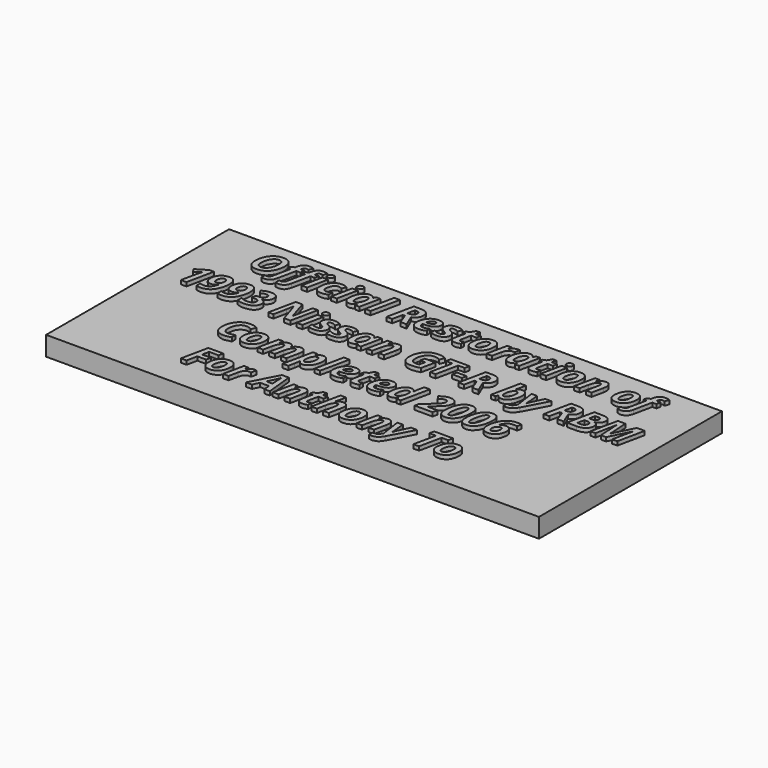
from build123d import *

# Parameters (mm, degrees)
F0_TEXT_SIZE = 12.5242310919
F2_DEPTH     = 7.62
F1_W         = 162.3541414738
F1_H         = 75.3404442221
F3_DEPTH     = 6.35


# Not quite as in the source:
# - Text() gives the source's letters only with a copy of the font that has no kerning and outlines rounded to 1/6400 em; it was checked with that copy


with BuildPart() as f2:
    # F0 (on Top) → F2 (new body)
    with BuildSketch(Plane.XY):
        with Locations((-64.2444132238, 17.4707429373)):
            Text('Official Restoration of', F0_TEXT_SIZE, font='Open Sans', font_style=FontStyle.BOLDITALIC, text_align=(TextAlign.LEFT, TextAlign.BOTTOM))
        with Locations((-74.0074427422, 0.4377886522)):
            Text('1993 Nissan GT-R by RBM', F0_TEXT_SIZE, font='Open Sans', font_style=FontStyle.BOLDITALIC, text_align=(TextAlign.LEFT, TextAlign.BOTTOM))
        with Locations((-47.9726973599, -16.5951656328)):
            Text('Completed 2006', F0_TEXT_SIZE, font='Open Sans', font_style=FontStyle.BOLDITALIC, text_align=(TextAlign.LEFT, TextAlign.BOTTOM))
        with Locations((-44.7183541871, -33.6281199178)):
            Text('For Anthony To', F0_TEXT_SIZE, font='Open Sans', font_style=FontStyle.BOLDITALIC, text_align=(TextAlign.LEFT, TextAlign.BOTTOM))
    extrude(amount=F2_DEPTH)


with BuildPart() as f3:
    # F1 (on Top) → F3 (new body)
    with BuildSketch(Plane.XY):
        with Locations((0, -5.4765110835)):
            Rectangle(F1_W, F1_H)
    extrude(amount=F3_DEPTH)


solid = Compound([f2.part, f3.part])
